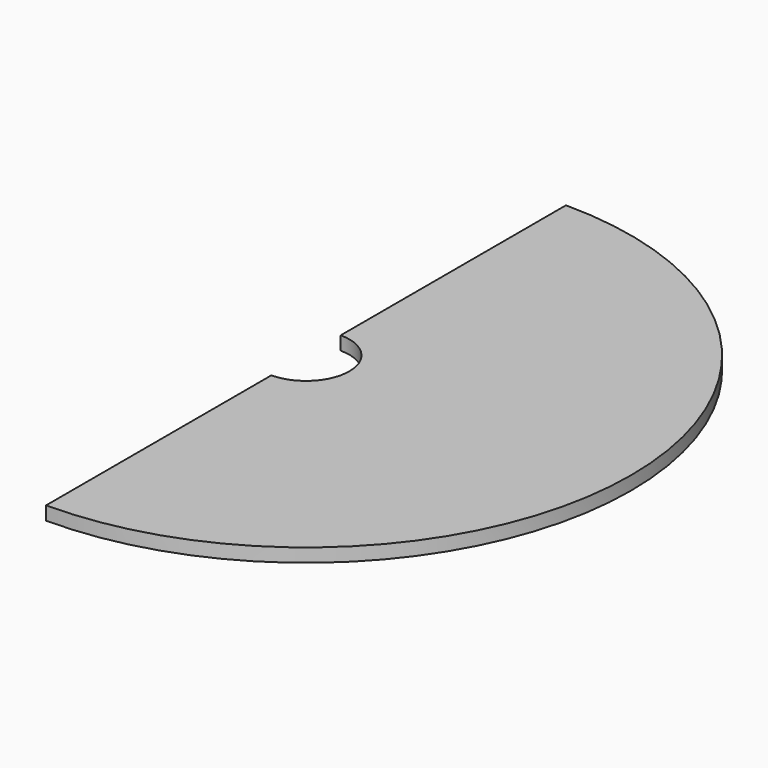
from build123d import *

# Parameters (mm, degrees)
F1_DEPTH = 5


# Not quite as in the source:
# - a feature names something its author has since deleted; it is built from what else it names


with BuildPart() as f1:
    # F0 (on Top) → F1 (new body)
    with BuildSketch(Plane.XY):
        with BuildLine():
            Line((0, -16), (0, -120))
            ThreePointArc((0, -120), (120, 0), (0, 120))
            Line((0, 120), (0, 16))
            ThreePointArc((0, 16), (11.313708499, 11.313708499), (16, 0))
            ThreePointArc((16, 0), (11.313708499, -11.313708499), (0, -16))
        make_face()
    extrude(amount=F1_DEPTH)


solid = f1.part
